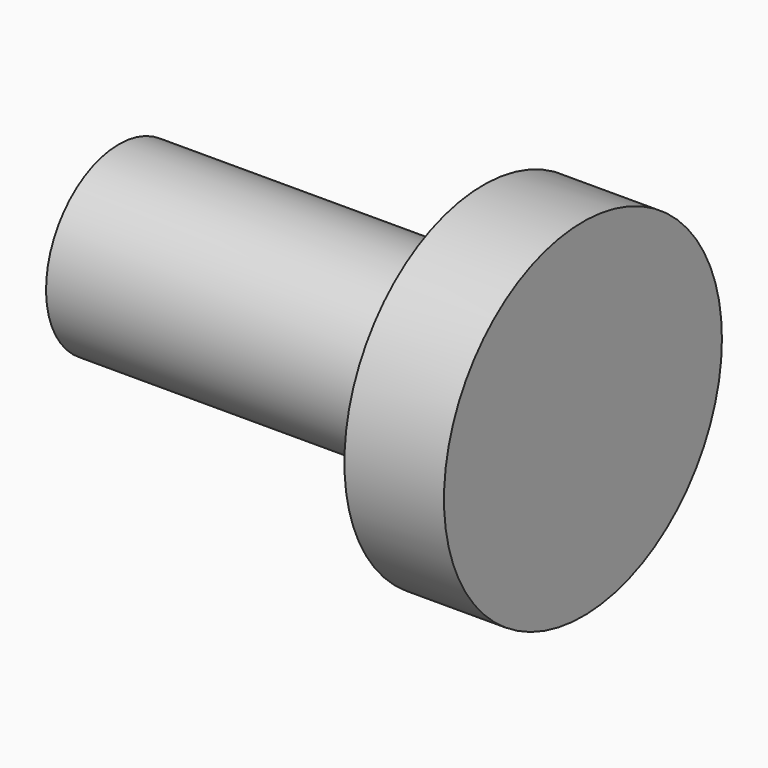
from build123d import *

# Parameters (mm, degrees)
F0_W     = 30
F0_H     = 7.5
F2_R     = 14.2998571377
F2_R_2   = 7.5
F3_DEPTH = 8.2


with BuildPart() as f1:
    # F0 (on Front) → F1 (revolve)
    with BuildSketch(Plane.XZ):
        with Locations((0, 3.75)):
            Rectangle(F0_W, F0_H)
    revolve(axis=Axis((0, 0, 0), (1, 0, 0)))

    # F2 (on face) → F3 (join)
    with BuildSketch(Plane.YZ.offset(15)):
        Circle(F2_R)
        Circle(F2_R_2, mode=Mode.SUBTRACT)
        Circle(F2_R_2)
    extrude(amount=F3_DEPTH)


solid = f1.part
